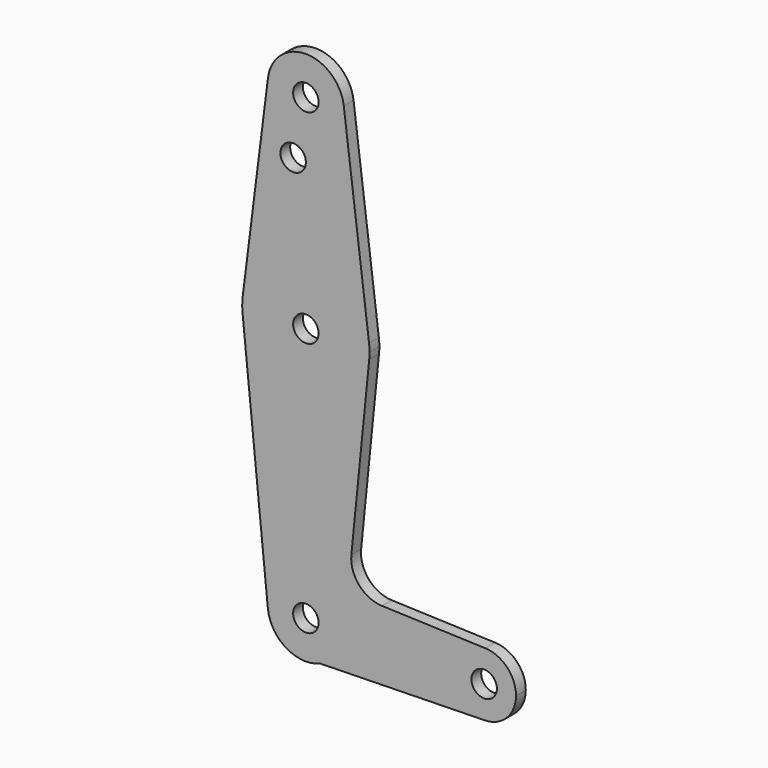
from build123d import *

# Parameters (mm, degrees)
F0_R     = 3.175
F1_DEPTH = 3.048


# Not quite as in the source:
# - a feature names something its author has since deleted; it is built from what else it names


with BuildPart() as f1:
    # F0 (on Front) → F1 (new body)
    with BuildSketch(Plane.XZ):
        with BuildLine():
            ThreePointArc((-9.4502929642, 115.490625), (-0.596483242, 104.7936951058), (9.525, 114.3))
            ThreePointArc((9.525, 114.3), (9.5063048942, 114.896483242), (9.4502929642, 115.490625))
            ThreePointArc((9.4502929642, 115.490625), (0, 123.825), (-9.4502929642, 115.490625))
        make_face()
        with Locations((0, 114.3)):
            Circle(F0_R, mode=Mode.SUBTRACT)
        with BuildLine():
            ThreePointArc((9.4502929642, 115.490625), (9.5063048942, 114.896483242), (9.525, 114.3))
            ThreePointArc((9.525, 114.3), (-0.596483242, 104.7936951058), (-9.4502929642, 115.490625))
            Line((-9.4502929642, 115.490625), (-15.7504882737, 65.484375))
            ThreePointArc((-15.7504882737, 65.484375), (0, 79.375), (15.7504882737, 65.484375))
            Line((15.7504882737, 65.484375), (9.4502929642, 115.490625))
        make_face()
        with Locations((-3.175, 100.0252)):
            Circle(F0_R, mode=Mode.SUBTRACT)
        with BuildLine():
            ThreePointArc((15.875, 63.5), (15.8438414904, 64.4941387366), (15.7504882737, 65.484375))
            ThreePointArc((15.7504882737, 65.484375), (0, 79.375), (-15.7504882737, 65.484375))
            ThreePointArc((-15.7504882737, 65.484375), (-15.8737438155, 63.6997054867), (-15.7954255641, 61.9125))
            ThreePointArc((-15.7954255641, 61.9125), (0, 47.625), (15.7954255641, 61.9125))
            ThreePointArc((15.7954255641, 61.9125), (15.8550939106, 62.7052534459), (15.875, 63.5))
        make_face()
        with Locations((0, 63.5)):
            Circle(F0_R, mode=Mode.SUBTRACT)
        with BuildLine():
            ThreePointArc((15.7954255641, 61.9125), (0, 47.625), (-15.7954255641, 61.9125))
            Line((-15.7954255641, 61.9125), (-9.4772553384, -0.9525))
            ThreePointArc((-9.4772553384, -0.9525), (-0.4768479324, 9.5130563464), (9.525, 0))
            ThreePointArc((9.525, 0), (7.9083579957, -5.3088133149), (3.6072049738, -8.8155372654))
            Line((3.6072049738, -8.8155372654), (44.6202460375, -7.9356740443))
            ThreePointArc((44.6202460375, -7.9356740443), (36.5127020955, 0.0566411934), (44.7334821429, 7.9324362036))
            Line((44.7334821429, 7.9324362036), (18.9676000005, 8.8532337108))
            ThreePointArc((18.9676000005, 8.8532337108), (13.2611998974, 11.5713591498), (11.3411865923, 17.5933818124))
            Line((11.3411865923, 17.5933818124), (15.7954255641, 61.9125))
        make_face()
        with BuildLine():
            ThreePointArc((9.525, 0), (-0.4768479324, 9.5130563464), (-9.4772553384, -0.9525))
            ThreePointArc((-9.4772553384, -0.9525), (-4.9062421037, -8.1642154197), (3.6072049738, -8.8155372654))
            ThreePointArc((3.6072049738, -8.8155372654), (7.9083579957, -5.3088133149), (9.525, 0))
        make_face()
        Circle(F0_R, mode=Mode.SUBTRACT)
        with BuildLine():
            ThreePointArc((44.7334821429, 7.9324362036), (36.5127020955, 0.0566411934), (44.6202460375, -7.9356740443))
            ThreePointArc((44.6202460375, -7.9356740443), (50.1225318057, -5.5521427543), (52.3875, 0))
            ThreePointArc((52.3875, 0), (50.1620069047, 5.5115227815), (44.7334821429, 7.9324362036))
        make_face()
        with Locations((44.45, 0)):
            Circle(F0_R, mode=Mode.SUBTRACT)
    extrude(amount=F1_DEPTH)


solid = f1.part
